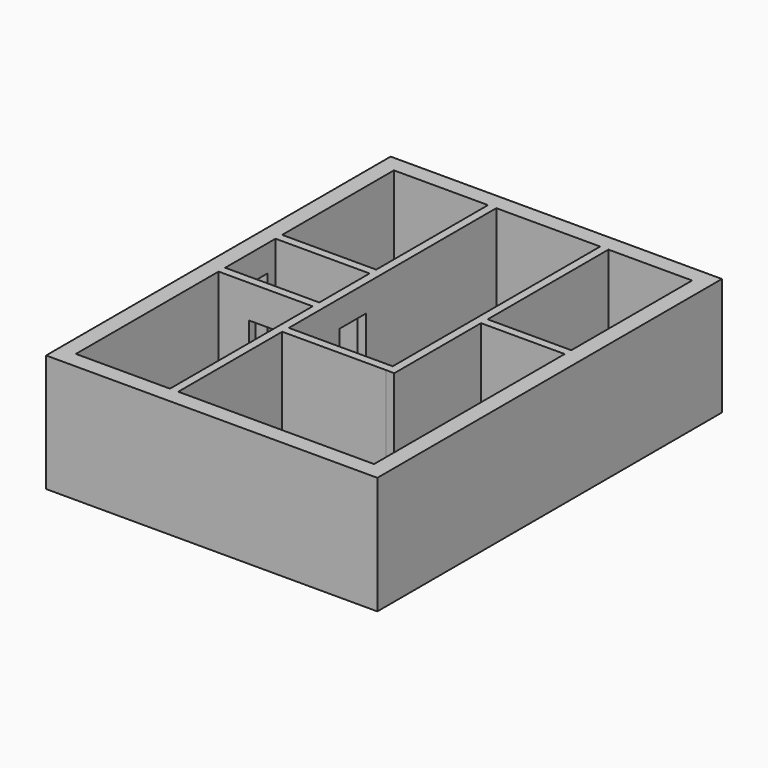
from build123d import *

# Parameters (mm, degrees)
F0_W      = 10000
F0_H      = 13000
F1_DEPTH  = 3550
F2_W      = 9000
F2_H      = 12000
F3_DEPTH  = 3300
F5_DEPTH  = 3300
F6_W      = 1000
F6_H      = 2300
F7_DEPTH  = 250
F8_W      = 1300
F8_H      = 2500
F9_DEPTH  = 21453
F10_W     = 1000
F10_H     = 2500
F11_DEPTH = 250
F12_W     = 3135.6891602224
F12_H     = 2800
F13_DEPTH = 250


# Not quite as in the source:
# - an extrude ends at something that could not be found from the text; its depth is read off the source's solid
# - a feature names something its author has since deleted; it is built from what else it names


with BuildPart() as f1:
    # F0 (on Top) → F1 (new body)
    with BuildSketch(Plane.XY):
        Rectangle(F0_W, F0_H)
    extrude(amount=F1_DEPTH)

    # F2 (on face) → F3 (cut)
    with BuildSketch(Plane.XY.offset(3550)):
        Rectangle(F2_W, F2_H)
    extrude(amount=-F3_DEPTH, mode=Mode.SUBTRACT)

    # F4 (on face) → F5 (join)
    with BuildSketch(Plane.XY.offset(250)):
        Polygon((-1660.4968309402, -366.6217029095), (-4500, -366.6217029095), (-4500, -616.6217029095), (-1660.4968309402, -616.6217029095), (-1660.4968309402, -6000), (-1410.4968309402, -6000), (-1410.4968309402, -2077.5351682588), (1725.1923292822, -2077.5351682588), (1975.1266148544, -2083.2669128011), (1975.1876689086, 1191.9026374817), (4500, 1191.9026374817), (4500, 1441.9026374817), (1975.1923292822, 1441.9026374817), (1975.1923292822, 6000), (1725.1923292822, 6000), (1725.1923292822, 1441.9026374817), (1725.1923292822, -1827.5351682588), (-1410.4968309402, -1827.5351682588), (-1410.4968309402, 6000), (-1660.4968309402, 6000), (-1660.4968309402, 1781.4515829086), (-4500, 1781.4515829086), (-4500, 1531.4515829086), (-1660.4968309402, 1531.4515829086), align=None)
    extrude(amount=F5_DEPTH)

    # F6 (on face) → F7 (cut)
    with BuildSketch(Plane.XZ.offset(616.6217029095)):
        with Locations((-3080.2484154701, 1400)):
            Rectangle(F6_W, F6_H)
    extrude(amount=-F7_DEPTH, mode=Mode.SUBTRACT)

    # F8 (on face) → F9 (cut, through all)
    with BuildSketch(Plane.YZ.offset(-4500)):
        with Locations((582.4149399996, 1500)):
            Rectangle(F8_W, F8_H)
    extrude(amount=-F9_DEPTH, mode=Mode.SUBTRACT)

    # F10 (on face) → F11 (cut, through all)
    with BuildSketch(Plane(origin=(-1660.4968309402, 0, 0), x_dir=(0, -1, 0), z_dir=(-1, 0, 0))):
        with Locations((-582.4149399996, 1500)):
            Rectangle(F10_W, F10_H)
    extrude(amount=-F11_DEPTH, mode=Mode.SUBTRACT)

    # F12 (on face) → F13 (cut, through all)
    with BuildSketch(Plane.XY.offset(250)):
        with Locations((157.347749171, 4600)):
            Rectangle(F12_W, F12_H)
    extrude(amount=-F13_DEPTH, mode=Mode.SUBTRACT)


solid = f1.part
